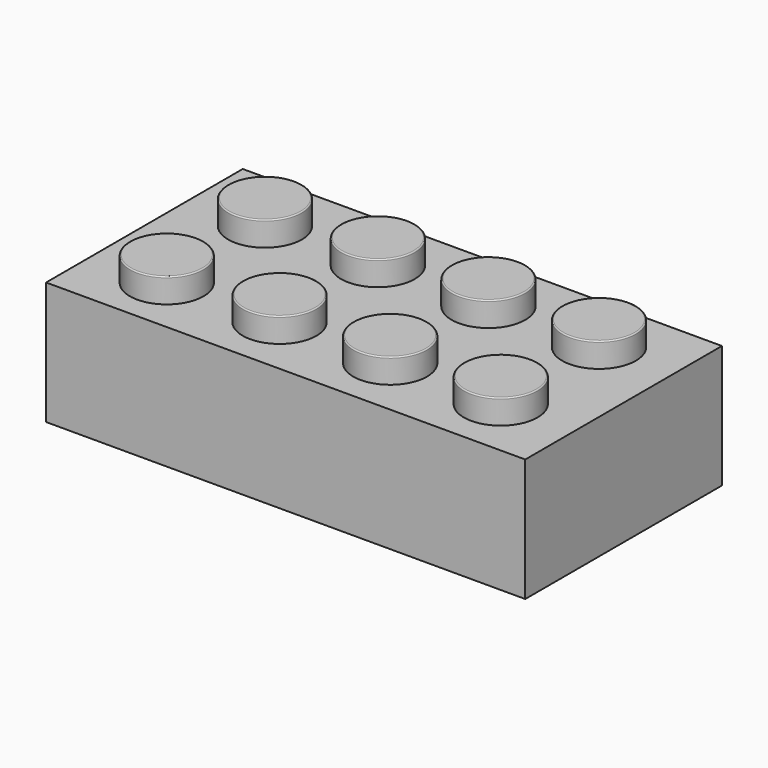
from build123d import *

# Parameters (mm, degrees)
F0_W      = 99.0672948342
F0_H      = 50.8267641079
F1_DEPTH  = 25.4
F2_R      = 7.626691027
F2_R_2    = 7.62
F3_DEPTH  = 5.08
F4_W      = 92.9712948342
F4_H      = 44.7307641079
F5_DEPTH  = 20.32
F7_DEPTH  = 15.24
F8_R      = 0.762
F9_DEPTH  = 15.24
F10_R     = 0.762
F6_R      = 9.906
F11_DEPTH = 20.32
F6_R_2    = 11.43
F6_W      = 2.032
F6_H      = 0.6096
F6_W_2    = 0.6096
F6_H_2    = 2.032
F6_W_3    = 0.611258532
F6_H_3    = 2.022552159
F6_H_4    = 2.0374442969
F12_R     = 0.508
F12_2_R   = 0.508
F12_3_R   = 0.508
F6_R_3    = 3.175
F13_DEPTH = 2.54
F14_R     = 0.254


# Not quite as in the source:
# - a feature names something its author has since deleted; it is built from what else it names


with BuildPart() as f1:
    # F0 (on Top) → F1 (new body)
    with BuildSketch(Plane.XY):
        with Locations((-3.7510339205, 0)):
            Rectangle(F0_W, F0_H)
    extrude(amount=F1_DEPTH)

    # F2 (on face) → F3 (join, symmetric)
    with BuildSketch(Plane.XY.offset(25.4)):
        with Locations((-15.1840765514, 12.706691027)):
            Circle(F2_R)
        with Locations((7.6826134967, 12.7)):
            Circle(F2_R_2)
        with Locations((30.5426134967, 12.7)):
            Circle(F2_R_2)
        with Locations((30.5426134967, -12.7)):
            Circle(F2_R_2)
        with Locations((7.6826134967, -12.7)):
            Circle(F2_R_2)
        with Locations((-15.1773865033, -12.7)):
            Circle(F2_R_2)
        with Locations((-38.0372540034, -13.2913871026)):
            Circle(F2_R_2)
        with Locations((-38.0429448591, 12.1086122599)):
            Circle(F2_R_2)
    extrude(amount=F3_DEPTH, both=True)

    # F4 (on face) → F5 (cut)
    with BuildSketch(Plane(origin=(0, 0, 0), x_dir=(1, 0, 0), z_dir=(0, 0, -1))):
        with Locations((-3.7510339205, 0)):
            Rectangle(F4_W, F4_H)
    extrude(amount=-F5_DEPTH, mode=Mode.SUBTRACT)

    # F6 (on face) → F7 (join)
    with BuildSketch(Plane(origin=(0, 0, 20.32), x_dir=(1, 0, 0), z_dir=(0, 0, -1))):
        with BuildLine():
            Line((-4.5616532358, -11.4044039181), (-4.5616532358, -22.3653820539))
            Line((-4.5616532358, -22.3653820539), (-3.0326388163, -22.3653820539))
            Line((-3.0326388163, -22.3653820539), (-3.0326388163, -11.4044039181))
            ThreePointArc((-3.0326388163, -11.4044039181), (-3.797146026, -11.43), (-4.5616532358, -11.4044039181))
        make_face()
    extrude(amount=F7_DEPTH)

    # F8
    f8_edges = [f1.edges().sort_by_distance(p)[0] for p in [
        (-3.032639, 16.884893, 5.08),
        (-4.561653, 16.884893, 5.08),
    ]]
    fillet(f8_edges, radius=F8_R)

    # F6 (on face) → F9 (join)
    with BuildSketch(Plane(origin=(0, 0, 20.32), x_dir=(1, 0, 0), z_dir=(0, 0, -1))):
        with BuildLine():
            Line((-4.5616532358, 22.3653820539), (-4.5616532358, 11.4044039181))
            ThreePointArc((-4.5616532358, 11.4044039181), (-3.797146026, 11.43), (-3.0326388163, 11.4044039181))
            Line((-3.0326388163, 11.4044039181), (-3.0326388163, 22.3653820539))
            Line((-3.0326388163, 22.3653820539), (-4.5616532358, 22.3653820539))
        make_face()
    extrude(amount=F9_DEPTH)

    # F10
    f10_edges = [f1.edges().sort_by_distance(p)[0] for p in [
        (-3.032639, -16.884893, 5.08),
        (-4.561653, -16.884893, 5.08),
    ]]
    fillet(f10_edges, radius=F10_R)

    # F6 (on face) → F13 (cut)
    with BuildSketch(Plane(origin=(0, 0, 20.32), x_dir=(1, 0, 0), z_dir=(0, 0, -1))):
        with Locations((34.302853974, -14.7453820539)):
            Circle(F6_R_3)
        with Locations((8.902853974, -14.7453820539)):
            Circle(F6_R_3)
        with Locations((8.902853974, 14.7453820539)):
            Circle(F6_R_3)
        with Locations((34.302853974, 14.7453820539)):
            Circle(F6_R_3)
        with Locations((-16.497146026, 14.7453820539)):
            Circle(F6_R_3)
        with Locations((-16.497146026, -14.7453820539)):
            Circle(F6_R_3)
        with Locations((-41.897146026, 14.7453820539)):
            Circle(F6_R_3)
        with Locations((-41.897146026, -14.7453820539)):
            Circle(F6_R_3)
    extrude(amount=-F13_DEPTH, mode=Mode.SUBTRACT)

    # F14
    f14_edges = [f1.edges().sort_by_distance(p)[0] for p in [
        (-22.797387, -12.7, 30.48),
        (0.062613, -12.7, 30.48),
        (22.922613, -12.7, 30.48),
        (22.922613, 12.7, 30.48),
        (0.062613, 12.7, 30.48),
        (-22.810768, 12.706691, 30.48),
        (-45.662945, 12.108612, 30.48),
        (-45.657254, -13.291387, 30.48),
    ]]
    fillet(f14_edges, radius=F14_R)


with BuildPart() as f11:
    # F6 (on face) → F11 (new body)
    with BuildSketch(Plane(origin=(0, 0, 20.32), x_dir=(1, 0, 0), z_dir=(0, 0, -1))):
        with BuildLine():
            ThreePointArc((-4.5616532358, 11.4044039181), (-15.227146026, 0), (-4.5616532358, -11.4044039181))
            ThreePointArc((-4.5616532358, -11.4044039181), (-3.797146026, -11.43), (-3.0326388163, -11.4044039181))
            ThreePointArc((-3.0326388163, -11.4044039181), (4.5510039908, -7.8072588849), (7.632853974, 0))
            ThreePointArc((7.632853974, 0), (4.5510039908, 7.8072588849), (-3.0326388163, 11.4044039181))
            ThreePointArc((-3.0326388163, 11.4044039181), (-3.797146026, 11.43), (-4.5616532358, 11.4044039181))
        make_face()
        with Locations((-3.797146026, 0)):
            Circle(F6_R, mode=Mode.SUBTRACT)
    extrude(amount=F11_DEPTH)

    # F12
    f12_edges = [f11.edges().sort_by_distance(p)[0] for p in [
        (-3.032639, -11.404404, 0),
        (-13.703146, 0, 0),
    ]]
    fillet(f12_edges, radius=F12_R)


with BuildPart() as f11b:
    # F6 (on face) → F11, piece 2 (new body)
    with BuildSketch(Plane(origin=(0, 0, 20.32), x_dir=(1, 0, 0), z_dir=(0, 0, -1))):
        with Locations((-29.197146026, 0)):
            Circle(F6_R_2)
        with Locations((-29.197146026, 0)):
            Circle(F6_R, mode=Mode.SUBTRACT)
    extrude(amount=F11_DEPTH)

    # F12#2
    f12_2_edges = [f11b.edges().sort_by_distance(p)[0] for p in [
        (-40.627146, 0, 0),
        (-39.103146, 0, 0),
    ]]
    fillet(f12_2_edges, radius=F12_2_R)


with BuildPart() as f11c:
    # F6 (on face) → F11, piece 3 (new body)
    with BuildSketch(Plane(origin=(0, 0, 20.32), x_dir=(1, 0, 0), z_dir=(0, 0, -1))):
        with Locations((21.602853974, 0)):
            Circle(F6_R_2)
        with Locations((21.602853974, 0)):
            Circle(F6_R, mode=Mode.SUBTRACT)
    extrude(amount=F11_DEPTH)

    # F12#3
    f12_3_edges = [f11c.edges().sort_by_distance(p)[0] for p in [
        (10.172854, 0, 0),
        (11.696854, 0, 0),
    ]]
    fillet(f12_3_edges, radius=F12_3_R)


with BuildPart() as f11d:
    # F6 (on face) → F11, piece 4 (new body)
    with BuildSketch(Plane(origin=(0, 0, 20.32), x_dir=(1, 0, 0), z_dir=(0, 0, -1))):
        with Locations((34.302853974, 22.0605820539)):
            Rectangle(F6_W, F6_H)
    extrude(amount=F11_DEPTH)


with BuildPart() as f11e:
    # F6 (on face) → F11, piece 5 (new body)
    with BuildSketch(Plane(origin=(0, 0, 20.32), x_dir=(1, 0, 0), z_dir=(0, 0, -1))):
        with Locations((42.4298134967, 14.7453820539)):
            Rectangle(F6_W_2, F6_H_2)
    extrude(amount=F11_DEPTH)


with BuildPart() as f11f:
    # F6 (on face) → F11, piece 6 (new body)
    with BuildSketch(Plane(origin=(0, 0, 20.32), x_dir=(1, 0, 0), z_dir=(0, 0, -1))):
        with Locations((42.4298134967, -14.7453820539)):
            Rectangle(F6_W_2, F6_H_2)
    extrude(amount=F11_DEPTH)


with BuildPart() as f11g:
    # F6 (on face) → F11, piece 7 (new body)
    with BuildSketch(Plane(origin=(0, 0, 20.32), x_dir=(1, 0, 0), z_dir=(0, 0, -1))):
        with Locations((34.302853974, -22.0605820539)):
            Rectangle(F6_W, F6_H)
    extrude(amount=F11_DEPTH)


with BuildPart() as f11h:
    # F6 (on face) → F11, piece 8 (new body)
    with BuildSketch(Plane(origin=(0, 0, 20.32), x_dir=(1, 0, 0), z_dir=(0, 0, -1))):
        with Locations((8.902853974, -22.0605820539)):
            Rectangle(F6_W, F6_H)
    extrude(amount=F11_DEPTH)


with BuildPart() as f11i:
    # F6 (on face) → F11, piece 9 (new body)
    with BuildSketch(Plane(origin=(0, 0, 20.32), x_dir=(1, 0, 0), z_dir=(0, 0, -1))):
        with Locations((-16.497146026, -22.0605820539)):
            Rectangle(F6_W, F6_H)
    extrude(amount=F11_DEPTH)


with BuildPart() as f11j:
    # F6 (on face) → F11, piece 10 (new body)
    with BuildSketch(Plane(origin=(0, 0, 20.32), x_dir=(1, 0, 0), z_dir=(0, 0, -1))):
        with Locations((-41.897146026, -22.0605820539)):
            Rectangle(F6_W, F6_H)
    extrude(amount=F11_DEPTH)


with BuildPart() as f11k:
    # F6 (on face) → F11, piece 11 (new body)
    with BuildSketch(Plane(origin=(0, 0, 20.32), x_dir=(1, 0, 0), z_dir=(0, 0, -1))):
        with Locations((-49.9310520716, -14.7453820539)):
            Rectangle(F6_W_3, F6_H_3)
    extrude(amount=F11_DEPTH)


with BuildPart() as f11l:
    # F6 (on face) → F11, piece 12 (new body)
    with BuildSketch(Plane(origin=(0, 0, 20.32), x_dir=(1, 0, 0), z_dir=(0, 0, -1))):
        with Locations((-49.9318813376, 14.7453820539)):
            Rectangle(F6_W_2, F6_H_4)
    extrude(amount=F11_DEPTH)


with BuildPart() as f11m:
    # F6 (on face) → F11, piece 13 (new body)
    with BuildSketch(Plane(origin=(0, 0, 20.32), x_dir=(1, 0, 0), z_dir=(0, 0, -1))):
        with Locations((-41.897146026, 22.0605820539)):
            Rectangle(F6_W, F6_H)
    extrude(amount=F11_DEPTH)


with BuildPart() as f11n:
    # F6 (on face) → F11, piece 14 (new body)
    with BuildSketch(Plane(origin=(0, 0, 20.32), x_dir=(1, 0, 0), z_dir=(0, 0, -1))):
        with Locations((-16.497146026, 22.0605820539)):
            Rectangle(F6_W, F6_H)
    extrude(amount=F11_DEPTH)


with BuildPart() as f11o:
    # F6 (on face) → F11, piece 15 (new body)
    with BuildSketch(Plane(origin=(0, 0, 20.32), x_dir=(1, 0, 0), z_dir=(0, 0, -1))):
        with Locations((8.902853974, 22.0605820539)):
            Rectangle(F6_W, F6_H)
    extrude(amount=F11_DEPTH)


solid = Compound([f1.part, f11.part, f11b.part, f11c.part, f11d.part, f11e.part, f11f.part, f11g.part, f11h.part, f11i.part, f11j.part, f11k.part, f11l.part, f11m.part, f11n.part, f11o.part])
